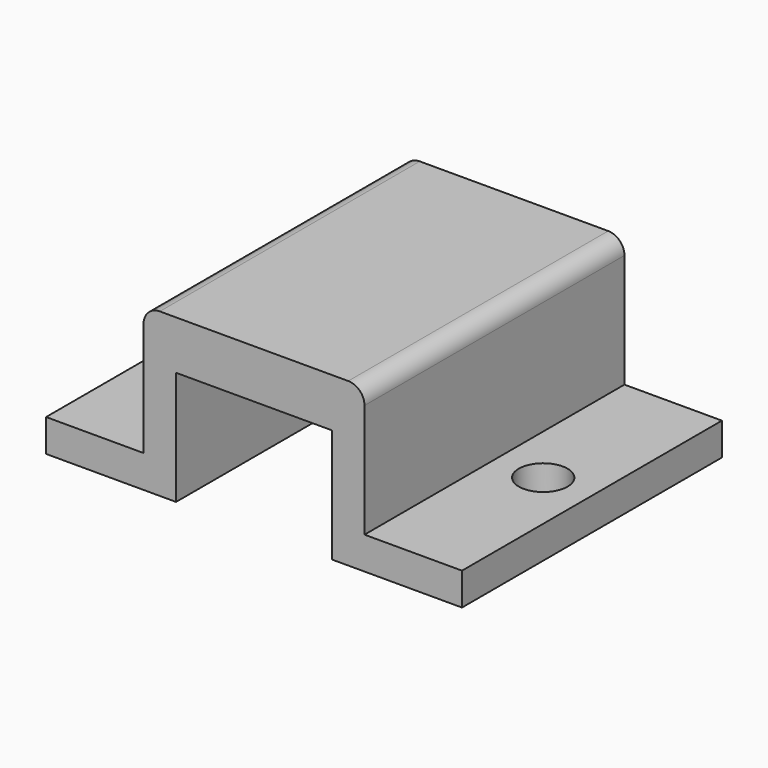
from build123d import *

# Parameters (mm, degrees)
F2_DEPTH = 25.4
F3_W     = 14.732
F3_H     = 0.635
F4_DEPTH = 3.81
F6_DEPTH = 3.81
F7_D     = 3.81


# Not quite as in the source:
# - a feature of the source that left no trace in its solid (it failed there, or was rolled back) is left out
# - a feature names something its author has since deleted; it is built from what else it names


with BuildPart() as f2:
    # F1 (on Front) → F2 (new body)
    with BuildSketch(Plane.XZ):
        with BuildLine():
            Line((-4.826, 5.08), (4.826, 5.08))
            ThreePointArc((4.826, 5.08), (5.7240256121, 4.7080256121), (6.096, 3.81))
            Line((6.096, 3.81), (6.096, -5.08))
            Line((6.096, -5.08), (16.256, -5.08))
            Line((16.256, -5.08), (16.256, -2.54))
            Line((16.256, -2.54), (8.636, -2.54))
            Line((8.636, -2.54), (8.636, 6.35))
            ThreePointArc((8.636, 6.35), (8.2640256121, 7.2480256121), (7.366, 7.62))
            Line((7.366, 7.62), (-7.366, 7.62))
            ThreePointArc((-7.366, 7.62), (-8.2640256121, 7.2480256121), (-8.636, 6.35))
            Line((-8.636, 6.35), (-8.636, -2.54))
            Line((-8.636, -2.54), (-16.256, -2.54))
            Line((-16.256, -2.54), (-16.256, -5.08))
            Line((-16.256, -5.08), (-6.096, -5.08))
            Line((-6.096, -5.08), (-6.096, 3.81))
            ThreePointArc((-6.096, 3.81), (-5.7240256121, 4.7080256121), (-4.826, 5.08))
        make_face()
    extrude(amount=F2_DEPTH)

    # F3 (on face) → F4 (join)
    with BuildSketch(Plane.XY.offset(7.62)):
        with Locations((0, -0.3175)):
            Rectangle(F3_W, F3_H)
    extrude(amount=-F4_DEPTH)

    # F3 (on face) → F6 (join)
    with BuildSketch(Plane.XY.offset(7.62)):
        with Locations((0, -25.0825)):
            Rectangle(F3_W, F3_H)
    extrude(amount=-F6_DEPTH)

    # F7 (through all)
    with Locations(Plane.XY.offset(-2.54)):
        with Locations((-12.446, -12.7), (12.446, -12.7)):
            Hole(F7_D / 2)


solid = f2.part
